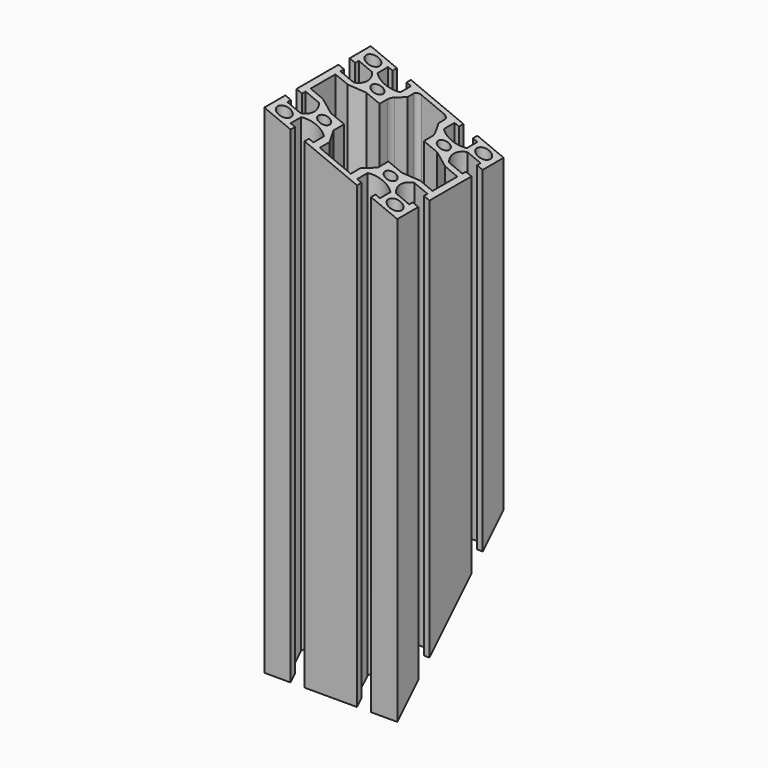
from build123d import *

# Parameters (mm, degrees)
F0_R          = 3
F0_R_2        = 2.5
F1_DEPTH      = 224.6
F2_R          = 2
F3_R          = 7
F6_DEPTH      = 30
F6_DEPTH_BACK = 30
F8_DEPTH      = 30
F8_DEPTH_BACK = 30


# Not quite as in the source:
# - a feature names something its author has since deleted; it is built from what else it names


with BuildPart() as f1:
    # F0 (on Top) → F1 (new body)
    with BuildSketch(Plane.XY):
        with BuildLine():
            Line((18.15, -30), (30, -30))
            Line((30, -30), (30, -18.15))
            Line((30, -18.15), (27.5, -18.15))
            Line((27.5, -18.15), (27.5, -20.15))
            Line((27.5, -20.15), (21.5477069044, -20.15))
            ThreePointArc((21.5477069044, -20.15), (19.5, -15), (21.5477069044, -9.85))
            Line((21.5477069044, -9.85), (27.5, -9.85))
            Line((27.5, -9.85), (27.5, -11.85))
            Line((27.5, -11.85), (30, -11.85))
            Line((30, -11.85), (30, 11.85))
            Line((30, 11.85), (27.5, 11.85))
            Line((27.5, 11.85), (27.5, 9.85))
            Line((27.5, 9.85), (21.5477069044, 9.85))
            ThreePointArc((21.5477069044, 9.85), (19.5, 15), (21.5477069044, 20.15))
            Line((21.5477069044, 20.15), (27.5, 20.15))
            Line((27.5, 20.15), (27.5, 18.15))
            Line((27.5, 18.15), (30, 18.15))
            Line((30, 18.15), (30, 30))
            Line((30, 30), (18.15, 30))
            Line((18.15, 30), (18.15, 27.5))
            Line((18.15, 27.5), (20.15, 27.5))
            Line((20.15, 27.5), (20.15, 21.5477069044))
            ThreePointArc((20.15, 21.5477069044), (15, 19.5), (9.85, 21.5477069044))
            Line((9.85, 21.5477069044), (9.85, 27.5))
            Line((9.85, 27.5), (11.85, 27.5))
            Line((11.85, 27.5), (11.85, 30))
            Line((11.85, 30), (-11.85, 30))
            Line((-11.85, 30), (-11.85, 27.5))
            Line((-11.85, 27.5), (-9.85, 27.5))
            Line((-9.85, 27.5), (-9.85, 21.5477069044))
            ThreePointArc((-9.85, 21.5477069044), (-15, 19.5), (-20.15, 21.5477069044))
            Line((-20.15, 21.5477069044), (-20.15, 27.5))
            Line((-20.15, 27.5), (-18.15, 27.5))
            Line((-18.15, 27.5), (-18.15, 30))
            Line((-18.15, 30), (-30, 30))
            Line((-30, 30), (-30, 18.15))
            Line((-30, 18.15), (-27.5, 18.15))
            Line((-27.5, 18.15), (-27.5, 20.15))
            Line((-27.5, 20.15), (-21.5477069044, 20.15))
            ThreePointArc((-21.5477069044, 20.15), (-19.5, 15), (-21.5477069044, 9.85))
            Line((-21.5477069044, 9.85), (-27.5, 9.85))
            Line((-27.5, 9.85), (-27.5, 11.85))
            Line((-27.5, 11.85), (-30, 11.85))
            Line((-30, 11.85), (-30, -11.85))
            Line((-30, -11.85), (-27.5, -11.85))
            Line((-27.5, -11.85), (-27.5, -9.85))
            Line((-27.5, -9.85), (-21.5477069044, -9.85))
            ThreePointArc((-21.5477069044, -9.85), (-19.5, -15), (-21.5477069044, -20.15))
            Line((-21.5477069044, -20.15), (-27.5, -20.15))
            Line((-27.5, -20.15), (-27.5, -18.15))
            Line((-27.5, -18.15), (-30, -18.15))
            Line((-30, -18.15), (-30, -30))
            Line((-30, -30), (-18.15, -30))
            Line((-18.15, -30), (-18.15, -27.5))
            Line((-18.15, -27.5), (-20.15, -27.5))
            Line((-20.15, -27.5), (-20.15, -21.5477069044))
            ThreePointArc((-20.15, -21.5477069044), (-15, -19.5), (-9.85, -21.5477069044))
            Line((-9.85, -21.5477069044), (-9.85, -27.5))
            Line((-9.85, -27.5), (-11.85, -27.5))
            Line((-11.85, -27.5), (-11.85, -30))
            Line((-11.85, -30), (11.85, -30))
            Line((11.85, -30), (11.85, -27.5))
            Line((11.85, -27.5), (9.85, -27.5))
            Line((9.85, -27.5), (9.85, -21.5477069044))
            ThreePointArc((9.85, -21.5477069044), (15, -19.5), (20.15, -21.5477069044))
            Line((20.15, -21.5477069044), (20.15, -27.5))
            Line((20.15, -27.5), (18.15, -27.5))
            Line((18.15, -27.5), (18.15, -30))
        make_face()
        with Locations((-25, -25)):
            Circle(F0_R, mode=Mode.SUBTRACT)
        with Locations((-15, -15)):
            Circle(F0_R_2, mode=Mode.SUBTRACT)
        with Locations((25, -25)):
            Circle(F0_R, mode=Mode.SUBTRACT)
        with Locations((15, -15)):
            Circle(F0_R_2, mode=Mode.SUBTRACT)
        with Locations((-25, 25)):
            Circle(F0_R, mode=Mode.SUBTRACT)
        with Locations((-15, 15)):
            Circle(F0_R_2, mode=Mode.SUBTRACT)
        Polygon((-7, 22), (-7, 27.5), (0, 27.5), (7, 27.5), (7, 22), (10, 16), (10, 10), (16, 10), (22, 7), (27.5, 7), (27.5, 0), (27.5, -7), (22, -7), (16, -10), (10, -10), (10, -16), (7, -22), (7, -27.5), (0, -27.5), (-7, -27.5), (-7, -22), (-10, -16), (-10, -10), (-16, -10), (-22, -7), (-27.5, -7), (-27.5, 0), (-27.5, 7), (-22, 7), (-16, 10), (-10, 10), (-10, 16), align=None, mode=Mode.SUBTRACT)
        with Locations((15, 15)):
            Circle(F0_R_2, mode=Mode.SUBTRACT)
        with Locations((25, 25)):
            Circle(F0_R, mode=Mode.SUBTRACT)
    extrude(amount=F1_DEPTH)

    # F2
    f2_edges = [f1.edges().sort_by_distance(p)[0] for p in [
        (-7, 27.5, 112.3),
        (7, 27.5, 112.3),
    ]]
    fillet(f2_edges, radius=F2_R)

    # F3
    f3_edges = [f1.edges().sort_by_distance(p)[0] for p in [
        (-10, 16, 112.3),
        (10, 16, 112.3),
    ]]
    fillet(f3_edges, radius=F3_R)

    # F5 (on Right) → F6 (cut, two sides)
    with BuildSketch(Plane.YZ) as f6_sk:
        Polygon((70.3932136338, -100.3932136338), (211.6390804038, 40.8526531362), (111.24586677, 141.24586677), (-30, 0), align=None)
    extrude(amount=-F6_DEPTH, mode=Mode.SUBTRACT)
    extrude(f6_sk.sketch, amount=F6_DEPTH_BACK, mode=Mode.SUBTRACT)

    # F7 (on Front) → F8 (cut, two sides)
    with BuildSketch(Plane.XZ) as f8_sk:
        Polygon((136.0873846676, 331.4359196356), (32.0951359741, 374.5109194261), (-30, 224.6), (73.9922486935, 181.5250002095), align=None)
    extrude(amount=F8_DEPTH, mode=Mode.SUBTRACT)
    extrude(f8_sk.sketch, amount=-F8_DEPTH_BACK, mode=Mode.SUBTRACT)


solid = f1.part
